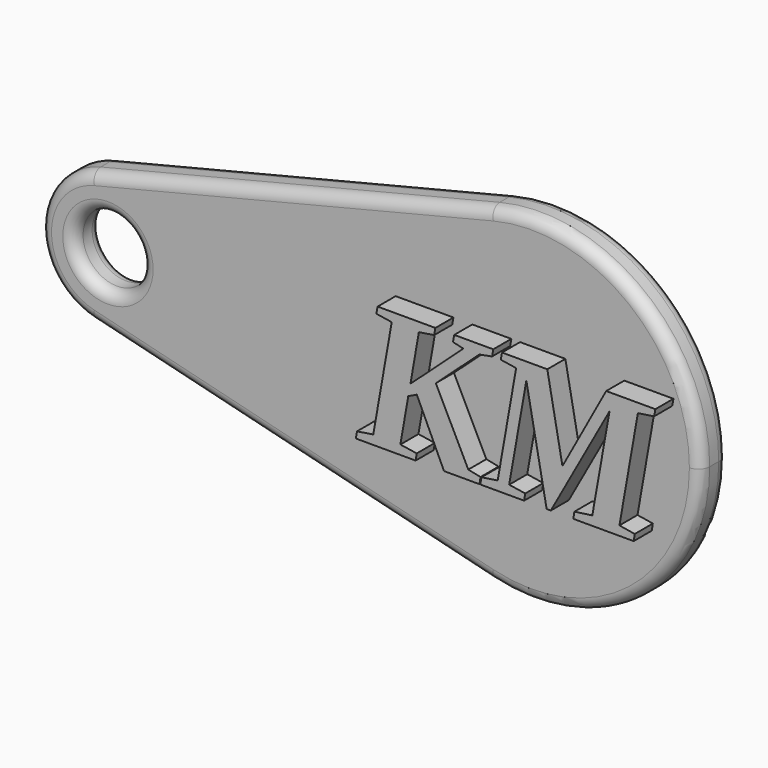
from build123d import *

# Parameters (mm, degrees)
F1_DEPTH     = 3
F2_TEXT_SIZE = 16.6663902959
F3_DEPTH     = 2
F4_R         = 3
F5_DEPTH     = 25
F6_R         = 1


# Not quite as in the source:
# - Text() gives the source's letters only with a copy of the font that has no kerning and outlines rounded to 1/6400 em; it was checked with that copy


with BuildPart() as f1:
    # F0 (on Front) → F1 (new body)
    with BuildSketch(Plane.XZ):
        with BuildLine():
            ThreePointArc((6.9279489781, -5.8246373278), (12.0665973798, -4.7244047244), (14.3679489781, 0))
            ThreePointArc((14.3679489781, 0), (12.0665973798, 4.7244047244), (6.9279489781, 5.8246373278))
            ThreePointArc((6.9279489781, 5.8246373278), (2.3679489781, 0), (6.9279489781, -5.8246373278))
        make_face()
        with BuildLine():
            ThreePointArc((6.9279489781, 5.8246373278), (12.0665973798, 4.7244047244), (14.3679489781, 0))
            ThreePointArc((14.3679489781, 0), (12.0665973798, -4.7244047244), (6.9279489781, -5.8246373278))
            Line((6.9279489781, -5.8246373278), (42.2679489781, -14.5615933194))
            ThreePointArc((42.2679489781, -14.5615933194), (30.8679489781, 0), (42.2679489781, 14.5615933194))
            Line((42.2679489781, 14.5615933194), (6.9279489781, 5.8246373278))
        make_face()
        with BuildLine():
            ThreePointArc((60.8679489781, 0), (55.1145699825, 11.811011811), (42.2679489781, 14.5615933194))
            ThreePointArc((42.2679489781, 14.5615933194), (30.8679489781, 0), (42.2679489781, -14.5615933194))
            ThreePointArc((42.2679489781, -14.5615933194), (55.1145699825, -11.811011811), (60.8679489781, 0))
        make_face()
    extrude(amount=F1_DEPTH)

    # F2 (on face) → F3 (join)
    with BuildSketch(Plane.XZ.offset(3)):
        with Locations((32.0510724097, -5.9999005065)):
            Text('KM', F2_TEXT_SIZE, font='Tinos', font_style=FontStyle.BOLDITALIC, text_align=(TextAlign.LEFT, TextAlign.BOTTOM))
    extrude(amount=F3_DEPTH)

    # F4 (on face) → F5 (cut)
    with BuildSketch(Plane.XZ.offset(3)):
        with Locations((8.3679489781, 0)):
            Circle(F4_R)
    extrude(amount=-F5_DEPTH, mode=Mode.SUBTRACT)

    # F6
    f6_edges = [f1.edges().sort_by_distance(p)[0] for p in [
        (24.597949, -3, 10.193115),
        (5.367949, -3, 0),
        (60.867949, 0, 0),
        (24.597949, 0, -10.193115),
        (2.367949, 0, 0),
        (60.867949, -3, 0),
        (24.597949, 0, 10.193115),
        (24.597949, -3, -10.193115),
        (2.367949, -3, 0),
        (5.367949, 0, 0),
    ]]
    fillet(f6_edges, radius=F6_R)


solid = f1.part
